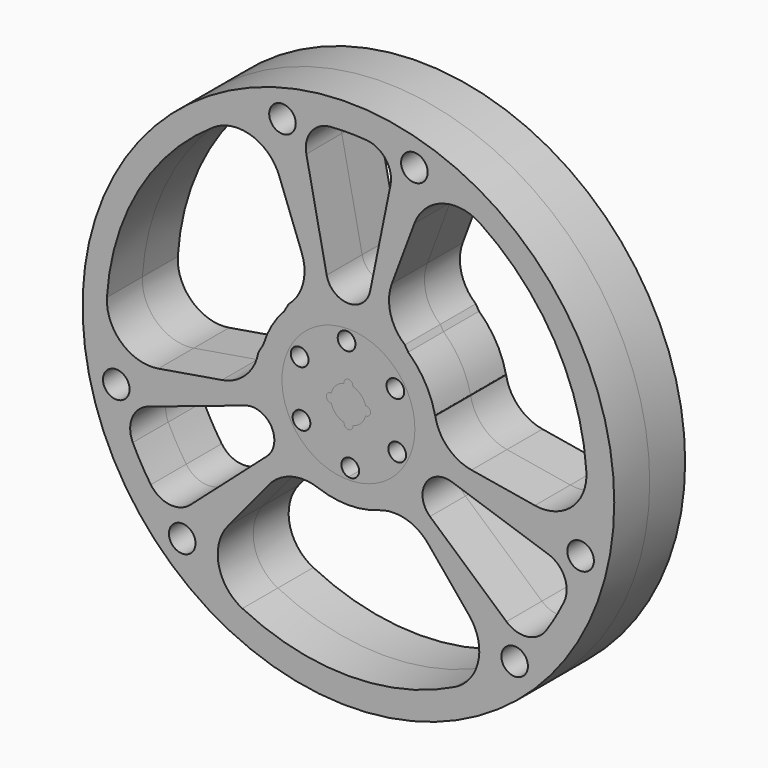
from build123d import *
from build123d import SkipClean  # not in build123d's __all__

# Parameters (mm, degrees)
F0_R     = 76.2
F1_DEPTH = 254
F2_DEPTH = 254
F0_R_2   = 50.8
F3_DEPTH = 254


with BuildPart() as f1:
    # F0 (on Front) → F1 (new body)
    with BuildSketch(Plane.XZ):
        with BuildLine():
            ThreePointArc((0, -1524), (1077.6307345283, -1077.6307345283), (1524, 0))
            ThreePointArc((1524, 0), (-1077.6307345283, 1077.6307345283), (0, -1524))
        make_face()
        with Locations((-952.7934209216, -986.6464701445)):
            Circle(F0_R, mode=Mode.SUBTRACT)
        with BuildLine():
            ThreePointArc((-905.9649252706, -801.5300581884), (-1025.7596879891, -838.6237549571), (-1132.816748196, -773.3128571327))
            ThreePointArc((-1132.816748196, -773.3128571327), (-1187.8404438307, -685.8), (-1236.116953448, -594.3916532038))
            ThreePointArc((-1236.116953448, -594.3916532038), (-1239.1493200045, -469.022070498), (-1147.1278549233, -383.8236111278))
            Line((-1147.1278549233, -383.8236111278), (-591.9672795655, -198.069481041))
            ThreePointArc((-591.9672795655, -198.069481041), (-441.6843619214, -255.0065852522), (-467.5168420786, -413.6239617924))
            Line((-467.5168420786, -413.6239617924), (-905.9649252706, -801.5300581884))
        make_face(mode=Mode.SUBTRACT)
        with Locations((-1330.8576181602, -331.8200720045)):
            Circle(F0_R, mode=Mode.SUBTRACT)
        with BuildLine():
            ThreePointArc((-456.9716264903, -554.3509110508), (-327.7273635176, -470.8420273415), (-173.9859882065, -477.2765193342))
            ThreePointArc((-173.9859882065, -477.2765193342), (0, -508), (173.9859882065, -477.2765193342))
            ThreePointArc((173.9859882065, -477.2765193342), (327.7273635176, -470.8420273415), (456.9716264903, -554.3509110508))
            Line((456.9716264903, -554.3509110508), (692.4035706036, -839.9526971225))
            ThreePointArc((692.4035706036, -839.9526971225), (744.8574525951, -1052.907398387), (611.380630262, -1226.9334091626))
            ThreePointArc((611.380630262, -1226.9334091626), (1.8222860374, -1370.1260113693), (-607.8626284159, -1227.4732811866))
            ThreePointArc((-607.8626284159, -1227.4732811866), (-743.4568649727, -1052.9960875563), (-691.0631281455, -838.3266103924))
            Line((-691.0631281455, -838.3266103924), (-456.9716264903, -554.3509110508))
        make_face(mode=Mode.SUBTRACT)
        with Locations((952.7934209216, -986.6464701445)):
            Circle(F0_R, mode=Mode.SUBTRACT)
        with BuildLine():
            ThreePointArc((1147.1278549233, -383.8236111278), (1239.1493200045, -469.022070498), (1236.116953448, -594.3916532039))
            ThreePointArc((1236.116953448, -594.3916532039), (1187.8404438307, -685.8), (1132.816748196, -773.3128571327))
            ThreePointArc((1132.816748196, -773.3128571327), (1025.7596879891, -838.6237549571), (905.9649252706, -801.5300581884))
            Line((905.9649252706, -801.5300581884), (467.5168420786, -413.6239617924))
            ThreePointArc((467.5168420786, -413.6239617924), (441.6843619214, -255.0065852522), (591.9672795655, -198.069481041))
            Line((591.9672795655, -198.069481041), (1147.1278549233, -383.8236111278))
        make_face(mode=Mode.SUBTRACT)
        with Locations((1330.8576181602, -331.8200720045)):
            Circle(F0_R, mode=Mode.SUBTRACT)
        with BuildLine():
            Line((-342.5097374141, 395.3599395107), (-369.4918522653, 348.6255456928))
            ThreePointArc((-369.4918522653, 348.6255456928), (-439.9409051225, 254), (-486.6645051108, 145.6765577067))
            Line((-486.6645051108, 145.6765577067), (-516.4957256206, 94.0073681319))
            ThreePointArc((-516.4957256206, 94.0073681319), (-587.7939797499, -42.3538144966), (-724.7369259702, -112.5281876697))
            Line((-724.7369259702, -112.5281876697), (-1089.7913001312, -173.6173390983))
            ThreePointArc((-1089.7913001312, -173.6173390983), (-1300.4424222774, -112.5663827978), (-1384.4149573618, 90.0409415469))
            ThreePointArc((-1384.4149573618, 90.0409415469), (-1203.6442163945, 689.5302538375), (-775.2608709103, 1146.2065129669))
            ThreePointArc((-775.2608709103, 1146.2065129669), (-556.3620705671, 1176.3959696166), (-396.6497183396, 1023.6869239431))
            Line((-396.6497183396, 1023.6869239431), (-267.76529948, 678.9698870289))
            ThreePointArc((-267.76529948, 678.9698870289), (-260.0666162324, 525.2866301464), (-342.5097374141, 395.3599395107))
        make_face(mode=Mode.SUBTRACT)
        with Locations((-378.0641972386, 1318.466542149)):
            Circle(F0_R, mode=Mode.SUBTRACT)
        with BuildLine():
            ThreePointArc((0, -381), (-269.4076836321, 269.4076836321), (381, 0))
            ThreePointArc((381, 0), (344.5974104181, -162.5226899025), (242.3458019258, -293.9889662707))
            ThreePointArc((242.3458019258, -293.9889662707), (128.7462695593, -358.5880618127), (0, -381))
        make_face(mode=Mode.SUBTRACT)
        with BuildLine():
            ThreePointArc((705.7186791676, -101.5479977586), (568.9475721526, -31.5438940564), (497.5617076924, 104.5111264482))
            ThreePointArc((497.5617076924, 104.5111264482), (497.3719004763, 104.4120103508), (497.1672799853, 104.3489133246))
            ThreePointArc((497.1672799853, 104.3489133246), (495.7725006908, 105.2563155454), (496.6782861088, 106.6521453514))
            ThreePointArc((496.6782861088, 106.6521453514), (440.5567920327, 252.9302532199), (342.5297761662, 375.1497733433))
            Line((342.5297761662, 375.1497733433), (323.4914906114, 406.3401294217))
            ThreePointArc((323.4914906114, 406.3401294217), (241.0483694297, 536.2668200575), (248.7470526773, 689.9500769399))
            Line((248.7470526773, 689.9500769399), (378.3694827249, 1036.6410144403))
            ThreePointArc((378.3694827249, 1036.6410144403), (536.5667228796, 1188.5447594043), (754.0160802971, 1159.9634458352))
            ThreePointArc((754.0160802971, 1159.9634458352), (1182.8036835544, 703.6667357513), (1364.1052525236, 104.3377464392))
            ThreePointArc((1364.1052525236, 104.3377464392), (1280.8006887371, -100.3289038409), (1068.6945996825, -162.2893353313))
            Line((1068.6945996825, -162.2893353313), (705.7186791676, -101.5479977586))
        make_face(mode=Mode.SUBTRACT)
        with BuildLine():
            ThreePointArc((-241.1629296527, 1185.3536693162), (-213.3896320154, 1307.6458254551), (-103.300205252, 1367.7045103365))
            ThreePointArc((-103.300205252, 1367.7045103365), (0, 1371.6), (103.300205252, 1367.7045103365))
            ThreePointArc((103.300205252, 1367.7045103365), (213.3896320154, 1307.6458254551), (241.1629296527, 1185.3536693162))
            Line((241.1629296527, 1185.3536693162), (124.4504374868, 611.6934428334))
            ThreePointArc((124.4504374868, 611.6934428334), (0, 510.0131705043), (-124.4504374868, 611.6934428334))
            Line((-124.4504374868, 611.6934428334), (-241.1629296527, 1185.3536693162))
        make_face(mode=Mode.SUBTRACT)
        with Locations((378.0641972386, 1318.466542149)):
            Circle(F0_R, mode=Mode.SUBTRACT)
    extrude(amount=F1_DEPTH)

    # F0 (on Front) → F2 (join, symmetric)
    with BuildSketch(Plane.XZ):
        with BuildLine():
            ThreePointArc((0, -1524), (1077.6307345283, -1077.6307345283), (1524, 0))
            ThreePointArc((1524, 0), (-1077.6307345283, 1077.6307345283), (0, -1524))
        make_face()
        with Locations((-952.7934209216, -986.6464701445)):
            Circle(F0_R, mode=Mode.SUBTRACT)
        with BuildLine():
            ThreePointArc((-905.9649252706, -801.5300581884), (-1025.7596879891, -838.6237549571), (-1132.816748196, -773.3128571327))
            ThreePointArc((-1132.816748196, -773.3128571327), (-1187.8404438307, -685.8), (-1236.116953448, -594.3916532038))
            ThreePointArc((-1236.116953448, -594.3916532038), (-1239.1493200045, -469.022070498), (-1147.1278549233, -383.8236111278))
            Line((-1147.1278549233, -383.8236111278), (-591.9672795655, -198.069481041))
            ThreePointArc((-591.9672795655, -198.069481041), (-441.6843619214, -255.0065852522), (-467.5168420786, -413.6239617924))
            Line((-467.5168420786, -413.6239617924), (-905.9649252706, -801.5300581884))
        make_face(mode=Mode.SUBTRACT)
        with Locations((-1330.8576181602, -331.8200720045)):
            Circle(F0_R, mode=Mode.SUBTRACT)
        with BuildLine():
            ThreePointArc((-456.9716264903, -554.3509110508), (-327.7273635176, -470.8420273415), (-173.9859882065, -477.2765193342))
            ThreePointArc((-173.9859882065, -477.2765193342), (0, -508), (173.9859882065, -477.2765193342))
            ThreePointArc((173.9859882065, -477.2765193342), (327.7273635176, -470.8420273415), (456.9716264903, -554.3509110508))
            Line((456.9716264903, -554.3509110508), (692.4035706036, -839.9526971225))
            ThreePointArc((692.4035706036, -839.9526971225), (744.8574525951, -1052.907398387), (611.380630262, -1226.9334091626))
            ThreePointArc((611.380630262, -1226.9334091626), (1.8222860374, -1370.1260113693), (-607.8626284159, -1227.4732811866))
            ThreePointArc((-607.8626284159, -1227.4732811866), (-743.4568649727, -1052.9960875563), (-691.0631281455, -838.3266103924))
            Line((-691.0631281455, -838.3266103924), (-456.9716264903, -554.3509110508))
        make_face(mode=Mode.SUBTRACT)
        with Locations((952.7934209216, -986.6464701445)):
            Circle(F0_R, mode=Mode.SUBTRACT)
        with BuildLine():
            ThreePointArc((1147.1278549233, -383.8236111278), (1239.1493200045, -469.022070498), (1236.116953448, -594.3916532039))
            ThreePointArc((1236.116953448, -594.3916532039), (1187.8404438307, -685.8), (1132.816748196, -773.3128571327))
            ThreePointArc((1132.816748196, -773.3128571327), (1025.7596879891, -838.6237549571), (905.9649252706, -801.5300581884))
            Line((905.9649252706, -801.5300581884), (467.5168420786, -413.6239617924))
            ThreePointArc((467.5168420786, -413.6239617924), (441.6843619214, -255.0065852522), (591.9672795655, -198.069481041))
            Line((591.9672795655, -198.069481041), (1147.1278549233, -383.8236111278))
        make_face(mode=Mode.SUBTRACT)
        with Locations((1330.8576181602, -331.8200720045)):
            Circle(F0_R, mode=Mode.SUBTRACT)
        with BuildLine():
            Line((-342.5097374141, 395.3599395107), (-369.4918522653, 348.6255456928))
            ThreePointArc((-369.4918522653, 348.6255456928), (-439.9409051225, 254), (-486.6645051108, 145.6765577067))
            Line((-486.6645051108, 145.6765577067), (-516.4957256206, 94.0073681319))
            ThreePointArc((-516.4957256206, 94.0073681319), (-587.7939797499, -42.3538144966), (-724.7369259702, -112.5281876697))
            Line((-724.7369259702, -112.5281876697), (-1089.7913001312, -173.6173390983))
            ThreePointArc((-1089.7913001312, -173.6173390983), (-1300.4424222774, -112.5663827978), (-1384.4149573618, 90.0409415469))
            ThreePointArc((-1384.4149573618, 90.0409415469), (-1203.6442163945, 689.5302538375), (-775.2608709103, 1146.2065129669))
            ThreePointArc((-775.2608709103, 1146.2065129669), (-556.3620705671, 1176.3959696166), (-396.6497183396, 1023.6869239431))
            Line((-396.6497183396, 1023.6869239431), (-267.76529948, 678.9698870289))
            ThreePointArc((-267.76529948, 678.9698870289), (-260.0666162324, 525.2866301464), (-342.5097374141, 395.3599395107))
        make_face(mode=Mode.SUBTRACT)
        with Locations((-378.0641972386, 1318.466542149)):
            Circle(F0_R, mode=Mode.SUBTRACT)
        with BuildLine():
            ThreePointArc((0, -381), (-269.4076836321, 269.4076836321), (381, 0))
            ThreePointArc((381, 0), (344.5974104181, -162.5226899025), (242.3458019258, -293.9889662707))
            ThreePointArc((242.3458019258, -293.9889662707), (128.7462695593, -358.5880618127), (0, -381))
        make_face(mode=Mode.SUBTRACT)
        with BuildLine():
            ThreePointArc((705.7186791676, -101.5479977586), (568.9475721526, -31.5438940564), (497.5617076924, 104.5111264482))
            ThreePointArc((497.5617076924, 104.5111264482), (497.3719004763, 104.4120103508), (497.1672799853, 104.3489133246))
            ThreePointArc((497.1672799853, 104.3489133246), (495.7725006908, 105.2563155454), (496.6782861088, 106.6521453514))
            ThreePointArc((496.6782861088, 106.6521453514), (440.5567920327, 252.9302532199), (342.5297761662, 375.1497733433))
            Line((342.5297761662, 375.1497733433), (323.4914906114, 406.3401294217))
            ThreePointArc((323.4914906114, 406.3401294217), (241.0483694297, 536.2668200575), (248.7470526773, 689.9500769399))
            Line((248.7470526773, 689.9500769399), (378.3694827249, 1036.6410144403))
            ThreePointArc((378.3694827249, 1036.6410144403), (536.5667228796, 1188.5447594043), (754.0160802971, 1159.9634458352))
            ThreePointArc((754.0160802971, 1159.9634458352), (1182.8036835544, 703.6667357513), (1364.1052525236, 104.3377464392))
            ThreePointArc((1364.1052525236, 104.3377464392), (1280.8006887371, -100.3289038409), (1068.6945996825, -162.2893353313))
            Line((1068.6945996825, -162.2893353313), (705.7186791676, -101.5479977586))
        make_face(mode=Mode.SUBTRACT)
        with BuildLine():
            ThreePointArc((-241.1629296527, 1185.3536693162), (-213.3896320154, 1307.6458254551), (-103.300205252, 1367.7045103365))
            ThreePointArc((-103.300205252, 1367.7045103365), (0, 1371.6), (103.300205252, 1367.7045103365))
            ThreePointArc((103.300205252, 1367.7045103365), (213.3896320154, 1307.6458254551), (241.1629296527, 1185.3536693162))
            Line((241.1629296527, 1185.3536693162), (124.4504374868, 611.6934428334))
            ThreePointArc((124.4504374868, 611.6934428334), (0, 510.0131705043), (-124.4504374868, 611.6934428334))
            Line((-124.4504374868, 611.6934428334), (-241.1629296527, 1185.3536693162))
        make_face(mode=Mode.SUBTRACT)
        with Locations((378.0641972386, 1318.466542149)):
            Circle(F0_R, mode=Mode.SUBTRACT)
    with SkipClean():  # cleaning this boolean's faces spoils the solid; the shape is the same uncleaned
        extrude(amount=F2_DEPTH, both=True)


with BuildPart() as f2:
    # F0 (on Front) → F2, piece 2 (new body, symmetric)
    with BuildSketch(Plane.XZ):
        with BuildLine():
            ThreePointArc((-25.2007812379, -98.425), (-19.05, -118.4005208253), (0, -127))
            ThreePointArc((0, -127), (19.05, -118.4005208253), (25.2007812379, -98.425))
            ThreePointArc((25.2007812379, -98.425), (71.8420489686, -71.8420489686), (98.425, -25.2007812379))
            ThreePointArc((98.425, -25.2007812379), (127, 0), (98.425, 25.2007812379))
            ThreePointArc((98.425, 25.2007812379), (71.8420489686, 71.8420489686), (25.2007812379, 98.425))
            ThreePointArc((25.2007812379, 98.425), (0, 127), (-25.2007812379, 98.425))
            ThreePointArc((-25.2007812379, 98.425), (-71.8420489686, 71.8420489686), (-98.425, 25.2007812379))
            ThreePointArc((-98.425, 25.2007812379), (-127, 0), (-98.425, -25.2007812379))
            ThreePointArc((-98.425, -25.2007812379), (-71.8420489686, -71.8420489686), (-25.2007812379, -98.425))
        make_face()
    extrude(amount=F2_DEPTH, both=True)


with BuildPart() as f3:
    # F0 (on Front) → F3 (new body)
    with BuildSketch(Plane.XZ):
        with BuildLine():
            ThreePointArc((242.3458019258, -293.9889662707), (344.5974104181, -162.5226899025), (381, 0))
            ThreePointArc((381, 0), (-269.4076836321, 269.4076836321), (0, -381))
            ThreePointArc((0, -381), (128.7462695593, -358.5880618127), (242.3458019258, -293.9889662707))
        make_face()
        with Locations((-269.1179451235, -167.6222195313)):
            Circle(F0_R_2, mode=Mode.SUBTRACT)
        with BuildLine():
            ThreePointArc((61.4061277911, -316.8740868568), (42.5580346842, -356.3673223016), (0, -366.5545664568))
            ThreePointArc((0, -366.5545664568), (-40.1938722089, -316.8740868568), (0, -267.1936072569))
            ThreePointArc((0, -267.1936072569), (42.5580346842, -277.3808514121), (61.4061277911, -316.8740868568))
        make_face(mode=Mode.SUBTRACT)
        with Locations((279.7240729146, -149.2518673255)):
            Circle(F0_R_2, mode=Mode.SUBTRACT)
        with Locations((-279.7240729146, 149.2518673255)):
            Circle(F0_R_2, mode=Mode.SUBTRACT)
        with Locations((-10.6061277911, 316.8740868568)):
            Circle(F0_R_2, mode=Mode.SUBTRACT)
        with BuildLine():
            ThreePointArc((25.2007812379, -98.425), (19.05, -118.4005208253), (0, -127))
            ThreePointArc((0, -127), (-19.05, -118.4005208253), (-25.2007812379, -98.425))
            ThreePointArc((-25.2007812379, -98.425), (-71.8420489686, -71.8420489686), (-98.425, -25.2007812379))
            ThreePointArc((-98.425, -25.2007812379), (-127, 0), (-98.425, 25.2007812379))
            ThreePointArc((-98.425, 25.2007812379), (-71.8420489686, 71.8420489686), (-25.2007812379, 98.425))
            ThreePointArc((-25.2007812379, 98.425), (0, 127), (25.2007812379, 98.425))
            ThreePointArc((25.2007812379, 98.425), (71.8420489686, 71.8420489686), (98.425, 25.2007812379))
            ThreePointArc((98.425, 25.2007812379), (127, 0), (98.425, -25.2007812379))
            ThreePointArc((98.425, -25.2007812379), (71.8420489686, -71.8420489686), (25.2007812379, -98.425))
        make_face(mode=Mode.SUBTRACT)
        with Locations((269.1179451235, 167.6222195313)):
            Circle(F0_R_2, mode=Mode.SUBTRACT)
    extrude(amount=F3_DEPTH)


solid = Compound([f1.part, f2.part, f3.part])
